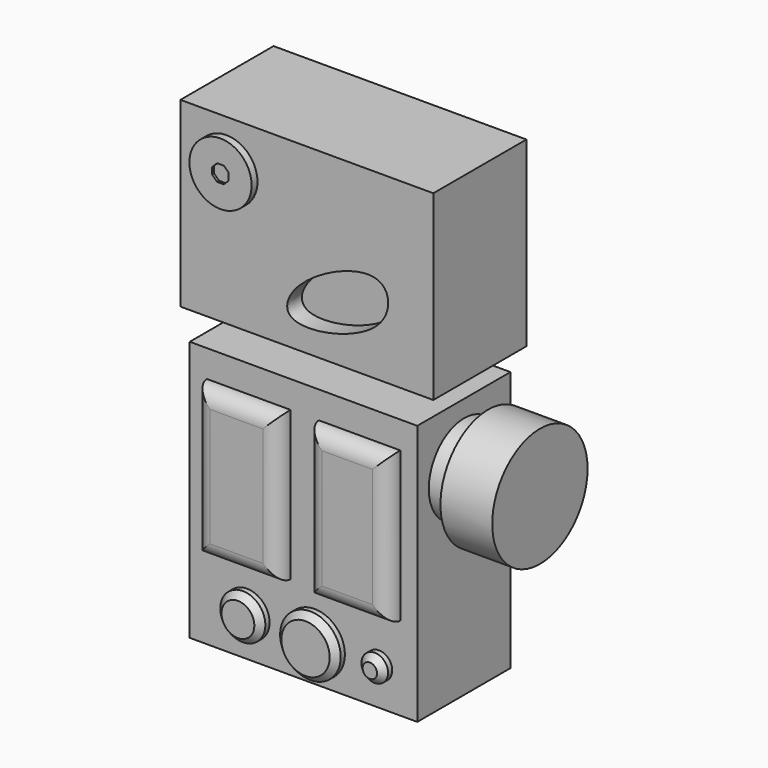
from build123d import *

# Parameters (mm, degrees)
F0_W      = 74.2475399747
F0_H      = 85.0587636232
F1_DEPTH  = 38
F2_W      = 27.2778645158
F2_H      = 48.6257560551
F2_W_2    = 26.5662674792
F2_H_2    = 48.8629546016
F3_DEPTH  = 5.1
F4_R      = 5
F5_R      = 7.356985616
F5_R_2    = 9.8858115492
F5_R_3    = 4.3495434343
F6_DEPTH  = 3.7
F7_SIZE   = 2
F8_R      = 14.4594029366
F9_DEPTH  = 7.8
F10_R     = 19.4422944141
F11_DEPTH = 16.9
F12_W     = 43.763179332
F12_H     = 9.2507535592
F13_DEPTH = 9.1
F14_W     = 82.5197082013
F14_H     = 37.9795394838
F15_DEPTH = 59.4
F17_DEPTH = 6
F18_R     = 10.1503328775
F19_DEPTH = 2.4
F21_DEPTH = 0.8


with BuildPart() as f1:
    # F0 (on Front) → F1 (new body)
    with BuildSketch(Plane.XZ):
        with Locations((-24.6077510528, -4.1337423027)):
            Rectangle(F0_W, F0_H)
    extrude(amount=F1_DEPTH)

    # F2 (on face) → F3 (join)
    with BuildSketch(Plane.XZ.offset(38)):
        with Locations((-42.4585863948, 5.2183736116)):
            Rectangle(F2_W, F2_H)
        with Locations((-6.2857677694, 5.0997743383)):
            Rectangle(F2_W_2, F2_H_2)
    extrude(amount=F3_DEPTH)

    # F4
    f4_edges = [f1.edges().sort_by_distance(p)[0] for p in [
        (-42.458586, -43.1, 29.531252),
        (-6.285768, -43.1, 29.531252),
        (-6.285768, -43.1, -19.331703),
        (-42.458586, -43.1, -19.094504),
        (-19.568902, -43.1, 5.099774),
        (-28.819654, -43.1, 5.218374),
        (-56.097519, -43.1, 5.218374),
        (6.997366, -43.1, 5.099774),
    ]]
    fillet(f4_edges, radius=F4_R)

    # F5 (on face) → F6 (join)
    with BuildSketch(Plane.XZ.offset(38)):
        with Locations((-43.0515818298, -33.8008292019)):
            Circle(F5_R)
        with Locations((-20.9920946509, -34.9868237972)):
            Circle(F5_R_2)
        with Locations((0, -34.5124267042)):
            Circle(F5_R_3)
    extrude(amount=F6_DEPTH)

    # F7
    f7_edges = [f1.edges().sort_by_distance(p)[0] for p in [
        (-50.408567, -41.7, -33.800829),
        (-30.877906, -41.7, -34.986824),
        (-4.349543, -41.7, -34.512427),
    ]]
    chamfer(f7_edges, length=F7_SIZE)

    # F8 (on face) → F9 (join)
    with BuildSketch(Plane.YZ.offset(12.5160189345)):
        with Locations((-18.8573058695, 18.3829069138)):
            Circle(F8_R)
    extrude(amount=F9_DEPTH)

    # F10 (on face) → F11 (join)
    with BuildSketch(Plane.YZ.offset(20.3160189345)):
        with Locations((-18.8573058695, 18.3829069138)):
            Circle(F10_R)
    extrude(amount=F11_DEPTH)

    # F12 (on face) → F13 (join)
    with BuildSketch(Plane.XY.offset(38.395639509)):
        with Locations((-21.881589666, -19.687501248)):
            Rectangle(F12_W, F12_H)
    extrude(amount=F13_DEPTH)

    # F14 (on face) → F15 (join)
    with BuildSketch(Plane.XY.offset(47.495639509)):
        with Locations((-23.5268557444, -18.9897697419)):
            Rectangle(F14_W, F14_H)
    extrude(amount=F15_DEPTH)

    # F16 (on face) → F17 (cut)
    with BuildSketch(Plane.XZ.offset(37.9795394838)):
        with BuildLine():
            add(Edge.make_bspline(
                [(-26.0310750455, 66.1403313279), (-19.5197759633, 72.7342236821), (3.3929896724, 82.8686218481), (4.6264940271, 58.9542461456), (-33.4389955915, 50.822229714), (-29.9990735288, 62.122000342), (-26.0310750455, 66.1403313279)],
                knots=[0, 0, 0, 0, 0.3027684682, 0.5046913629, 0.8154922992, 1, 1, 1, 1], degree=3))
        make_face()
    extrude(amount=-F17_DEPTH, mode=Mode.SUBTRACT)

    # F18 (on face) → F19 (join)
    with BuildSketch(Plane.XZ.offset(37.9795394838)):
        with Locations((-49.7975498438, 91.5002599359)):
            Circle(F18_R)
    extrude(amount=F19_DEPTH)

    # F20 (on face) → F21 (cut)
    with BuildSketch(Plane.XZ.offset(40.3795394838)):
        Polygon((-50.9105199745, 88.8133123517), (-48.684579713, 88.8133123517), (-47.1106022596, 90.3872898051), (-47.1106022596, 92.6132300666), (-48.684579713, 94.18720752), (-50.9105199745, 94.18720752), (-52.4844974279, 92.6132300666), (-52.4844974279, 90.3872898051), align=None)
    extrude(amount=-F21_DEPTH, mode=Mode.SUBTRACT)


solid = f1.part
